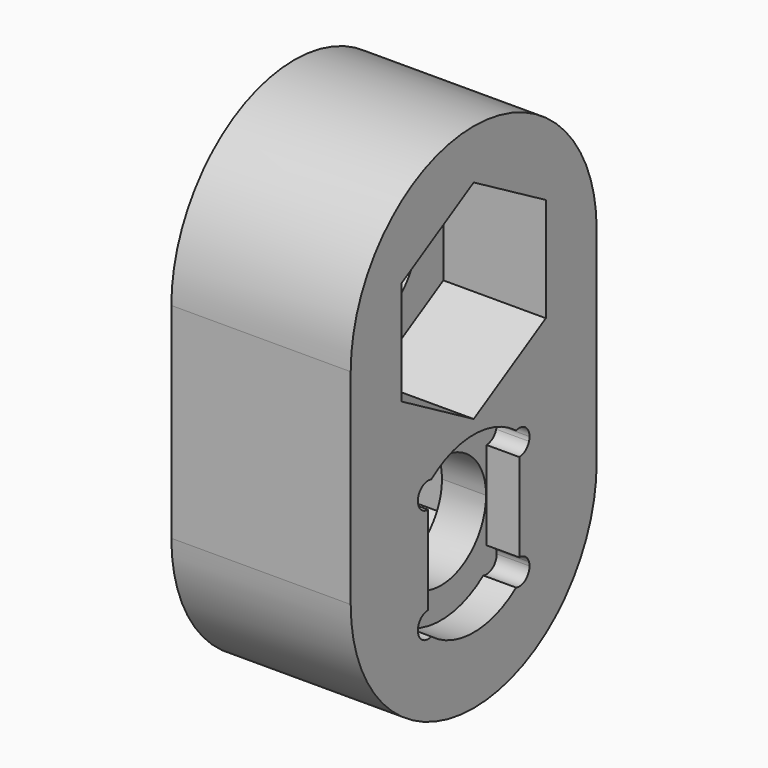
from build123d import *

# Parameters (mm, degrees)
F1_DEPTH = 5.55752
F2_R     = 1.75
F3_DEPTH = 1.016
F4_R     = 1.75
F5_DEPTH = 1.016
F6_DEPTH = 3.175
F7_DEPTH = 3.175


# Not quite as in the source:
# - a feature names something its author has since deleted; it is built from what else it names


with BuildPart() as f1:
    # F0 (on Right) → F1 (new body)
    with BuildSketch(Plane.YZ):
        with BuildLine():
            ThreePointArc((0.636344373, -4.7197957677), (2.2310225415, -4.2076055743), (3.5497579143, -3.175))
            ThreePointArc((3.5497579143, -3.175), (2.2310225415, -2.1423944257), (0.636344373, -1.6302042323))
            ThreePointArc((0.636344373, -1.6302042323), (0, -1.75), (-0.636344373, -1.6302042323))
            ThreePointArc((-0.636344373, -1.6302042323), (-2.2310225415, -2.1423944257), (-3.5497579143, -3.175))
            ThreePointArc((-3.5497579143, -3.175), (-2.2310225415, -4.2076055743), (-0.636344373, -4.7197957677))
            ThreePointArc((-0.636344373, -4.7197957677), (0, -4.6), (0.636344373, -4.7197957677))
        make_face()
        with BuildLine():
            ThreePointArc((3.5497579143, -3.175), (4.4489958596, -1.6993652025), (4.7625, 0))
            ThreePointArc((4.7625, 0), (0, 4.7625), (-4.7625, 0))
            ThreePointArc((-4.7625, 0), (-4.4489958596, -1.6993652025), (-3.5497579143, -3.175))
            ThreePointArc((-3.5497579143, -3.175), (-2.2310225415, -2.1423944257), (-0.636344373, -1.6302042323))
            ThreePointArc((-0.636344373, -1.6302042323), (-0.9871416685, 1.4450091094), (1.75, 0))
            ThreePointArc((1.75, 0), (1.4450091094, -0.9871416685), (0.636344373, -1.6302042323))
            ThreePointArc((0.636344373, -1.6302042323), (2.2310225415, -2.1423944257), (3.5497579143, -3.175))
        make_face()
        with BuildLine():
            Line((4.7625, -6.35), (4.7625, 0))
            ThreePointArc((4.7625, 0), (4.4489958596, -1.6993652025), (3.5497579143, -3.175))
            ThreePointArc((3.5497579143, -3.175), (4.4489958596, -4.6506347975), (4.7625, -6.35))
        make_face()
        with BuildLine():
            ThreePointArc((4.7625, -6.35), (4.4489958596, -4.6506347975), (3.5497579143, -3.175))
            ThreePointArc((3.5497579143, -3.175), (2.2310225415, -4.2076055743), (0.636344373, -4.7197957677))
            ThreePointArc((0.636344373, -4.7197957677), (1.4450091094, -5.3628583315), (1.75, -6.35))
            ThreePointArc((1.75, -6.35), (-0.9871416685, -7.7950091094), (-0.636344373, -4.7197957677))
            ThreePointArc((-0.636344373, -4.7197957677), (-2.2310225415, -4.2076055743), (-3.5497579143, -3.175))
            ThreePointArc((-3.5497579143, -3.175), (-4.4489958596, -4.6506347975), (-4.7625, -6.35))
            ThreePointArc((-4.7625, -6.35), (0, -11.1125), (4.7625, -6.35))
        make_face()
        with BuildLine():
            ThreePointArc((-3.5497579143, -3.175), (-4.4489958596, -1.6993652025), (-4.7625, 0))
            Line((-4.7625, 0), (-4.7625, -6.35))
            ThreePointArc((-4.7625, -6.35), (-4.4489958596, -4.6506347975), (-3.5497579143, -3.175))
        make_face()
    extrude(amount=F1_DEPTH)

    # F2 (on face) → F3 (cut)
    with BuildSketch(Plane.YZ.offset(5.55752)):
        with BuildLine():
            ThreePointArc((1.368425, -4.5847), (1.4846669962, -4.8653330038), (1.7653, -4.981575))
            Line((1.7653, -4.981575), (1.7653, -4.5847))
            Line((1.7653, -4.5847), (1.368425, -4.5847))
        make_face()
        with BuildLine():
            Line((1.7653, -4.5847), (1.7653, -4.981575))
            ThreePointArc((1.7653, -4.981575), (1.9986038099, -4.9057593371), (2.1427708235, -4.7072787218))
            ThreePointArc((2.1427708235, -4.7072787218), (1.9091883092, -4.4408116908), (1.6427212782, -4.2072291765))
            ThreePointArc((1.6427212782, -4.2072291765), (1.4442406629, -4.3513961901), (1.368425, -4.5847))
            Line((1.368425, -4.5847), (1.7653, -4.5847))
        make_face()
        with BuildLine():
            ThreePointArc((1.7653, -7.718425), (1.4846669962, -7.8346669962), (1.368425, -8.1153))
            Line((1.368425, -8.1153), (1.7653, -8.1153))
            Line((1.7653, -8.1153), (1.7653, -7.718425))
        make_face()
        with BuildLine():
            Line((1.7653, -8.1153), (1.368425, -8.1153))
            ThreePointArc((1.368425, -8.1153), (1.4442406629, -8.3486038099), (1.6427212782, -8.4927708235))
            ThreePointArc((1.6427212782, -8.4927708235), (1.9091883092, -8.2591883092), (2.1427708235, -7.9927212782))
            ThreePointArc((2.1427708235, -7.9927212782), (1.9986038099, -7.7942406629), (1.7653, -7.718425))
            Line((1.7653, -7.718425), (1.7653, -8.1153))
        make_face()
        with BuildLine():
            Line((-1.368425, -8.1153), (-1.7653, -8.1153))
            Line((-1.7653, -8.1153), (-1.7653, -7.718425))
            ThreePointArc((-1.7653, -7.718425), (-1.9986038099, -7.7942406629), (-2.1427708235, -7.9927212782))
            ThreePointArc((-2.1427708235, -7.9927212782), (-1.9091883092, -8.2591883092), (-1.6427212782, -8.4927708235))
            ThreePointArc((-1.6427212782, -8.4927708235), (-1.4442406629, -8.3486038099), (-1.368425, -8.1153))
        make_face()
        with BuildLine():
            Line((-1.7653, -7.718425), (-1.7653, -8.1153))
            Line((-1.7653, -8.1153), (-1.368425, -8.1153))
            ThreePointArc((-1.368425, -8.1153), (-1.4846669962, -7.8346669962), (-1.7653, -7.718425))
        make_face()
        with BuildLine():
            Line((-1.7653, -4.5847), (-1.7653, -4.981575))
            ThreePointArc((-1.7653, -4.981575), (-1.4846669962, -4.8653330038), (-1.368425, -4.5847))
            Line((-1.368425, -4.5847), (-1.7653, -4.5847))
        make_face()
        with BuildLine():
            ThreePointArc((-2.1427708235, -4.7072787218), (-1.9986038099, -4.9057593371), (-1.7653, -4.981575))
            Line((-1.7653, -4.981575), (-1.7653, -4.5847))
            Line((-1.7653, -4.5847), (-1.368425, -4.5847))
            ThreePointArc((-1.368425, -4.5847), (-1.4442406629, -4.3513961901), (-1.6427212782, -4.2072291765))
            ThreePointArc((-1.6427212782, -4.2072291765), (-1.9091883092, -4.4408116908), (-2.1427708235, -4.7072787218))
        make_face()
        with BuildLine():
            ThreePointArc((-1.7653, -7.718425), (-1.4846669962, -7.8346669962), (-1.368425, -8.1153))
            Line((-1.368425, -8.1153), (1.368425, -8.1153))
            ThreePointArc((1.368425, -8.1153), (1.4846669962, -7.8346669962), (1.7653, -7.718425))
            Line((1.7653, -7.718425), (1.7653, -4.981575))
            ThreePointArc((1.7653, -4.981575), (1.4846669962, -4.8653330038), (1.368425, -4.5847))
            Line((1.368425, -4.5847), (-1.368425, -4.5847))
            ThreePointArc((-1.368425, -4.5847), (-1.4846669962, -4.8653330038), (-1.7653, -4.981575))
            Line((-1.7653, -4.981575), (-1.7653, -7.718425))
        make_face()
        with Locations((0, -6.35)):
            Circle(F2_R, mode=Mode.SUBTRACT)
        with BuildLine():
            ThreePointArc((-1.6427212782, -4.2072291765), (-2.0459330038, -4.3040669962), (-2.1427708235, -4.7072787218))
            ThreePointArc((-2.1427708235, -4.7072787218), (-1.9091883092, -4.4408116908), (-1.6427212782, -4.2072291765))
        make_face()
        with BuildLine():
            ThreePointArc((1.6427212782, -4.2072291765), (1.9091883092, -4.4408116908), (2.1427708235, -4.7072787218))
            ThreePointArc((2.1427708235, -4.7072787218), (2.1572939405, -4.6467525283), (2.162175, -4.5847))
            ThreePointArc((2.162175, -4.5847), (1.9986038099, -4.2636406629), (1.6427212782, -4.2072291765))
        make_face()
        with BuildLine():
            ThreePointArc((2.1427708235, -7.9927212782), (1.9091883092, -8.2591883092), (1.6427212782, -8.4927708235))
            ThreePointArc((1.6427212782, -8.4927708235), (1.9986038099, -8.4363593371), (2.162175, -8.1153))
            ThreePointArc((2.162175, -8.1153), (2.1572939405, -8.0532474717), (2.1427708235, -7.9927212782))
        make_face()
        with BuildLine():
            ThreePointArc((-2.1427708235, -7.9927212782), (-2.0459330038, -8.3959330038), (-1.6427212782, -8.4927708235))
            ThreePointArc((-1.6427212782, -8.4927708235), (-1.9091883092, -8.2591883092), (-2.1427708235, -7.9927212782))
        make_face()
        with BuildLine():
            ThreePointArc((-1.6427212782, -4.2072291765), (-1.4442406629, -4.3513961901), (-1.368425, -4.5847))
            Line((-1.368425, -4.5847), (1.368425, -4.5847))
            ThreePointArc((1.368425, -4.5847), (1.4442406629, -4.3513961901), (1.6427212782, -4.2072291765))
            ThreePointArc((1.6427212782, -4.2072291765), (0, -3.65), (-1.6427212782, -4.2072291765))
        make_face()
        with BuildLine():
            Line((1.368425, -8.1153), (-1.368425, -8.1153))
            ThreePointArc((-1.368425, -8.1153), (-1.4442406629, -8.3486038099), (-1.6427212782, -8.4927708235))
            ThreePointArc((-1.6427212782, -8.4927708235), (0, -9.05), (1.6427212782, -8.4927708235))
            ThreePointArc((1.6427212782, -8.4927708235), (1.4442406629, -8.3486038099), (1.368425, -8.1153))
        make_face()
    extrude(amount=-F3_DEPTH, mode=Mode.SUBTRACT)

    # F4 (on face) → F5 (cut)
    with BuildSketch(Plane(origin=(0, 0, 0), x_dir=(0, -1, 0), z_dir=(-1, 0, 0))):
        with BuildLine():
            ThreePointArc((1.7653, -1.368425), (1.4846669962, -1.4846669962), (1.368425, -1.7653))
            Line((1.368425, -1.7653), (1.7653, -1.7653))
            Line((1.7653, -1.7653), (1.7653, -1.368425))
        make_face()
        with BuildLine():
            Line((1.7653, -1.7653), (1.368425, -1.7653))
            ThreePointArc((1.368425, -1.7653), (1.4442406629, -1.9986038099), (1.6427212782, -2.1427708235))
            ThreePointArc((1.6427212782, -2.1427708235), (1.9091883092, -1.9091883092), (2.1427708235, -1.6427212782))
            ThreePointArc((2.1427708235, -1.6427212782), (1.9986038099, -1.4442406629), (1.7653, -1.368425))
            Line((1.7653, -1.368425), (1.7653, -1.7653))
        make_face()
        with BuildLine():
            Line((-1.7653, -1.368425), (-1.7653, -1.7653))
            Line((-1.7653, -1.7653), (-1.368425, -1.7653))
            ThreePointArc((-1.368425, -1.7653), (-1.4846669962, -1.4846669962), (-1.7653, -1.368425))
        make_face()
        with BuildLine():
            Line((-1.368425, -1.7653), (-1.7653, -1.7653))
            Line((-1.7653, -1.7653), (-1.7653, -1.368425))
            ThreePointArc((-1.7653, -1.368425), (-1.9986038099, -1.4442406629), (-2.1427708235, -1.6427212782))
            ThreePointArc((-2.1427708235, -1.6427212782), (-1.9091883092, -1.9091883092), (-1.6427212782, -2.1427708235))
            ThreePointArc((-1.6427212782, -2.1427708235), (-1.4442406629, -1.9986038099), (-1.368425, -1.7653))
        make_face()
        with BuildLine():
            Line((-1.7653, 1.7653), (-1.7653, 1.368425))
            ThreePointArc((-1.7653, 1.368425), (-1.4846669962, 1.4846669962), (-1.368425, 1.7653))
            Line((-1.368425, 1.7653), (-1.7653, 1.7653))
        make_face()
        with BuildLine():
            ThreePointArc((-2.1427708235, 1.6427212782), (-1.9986038099, 1.4442406629), (-1.7653, 1.368425))
            Line((-1.7653, 1.368425), (-1.7653, 1.7653))
            Line((-1.7653, 1.7653), (-1.368425, 1.7653))
            ThreePointArc((-1.368425, 1.7653), (-1.4442406629, 1.9986038099), (-1.6427212782, 2.1427708235))
            ThreePointArc((-1.6427212782, 2.1427708235), (-1.9091883092, 1.9091883092), (-2.1427708235, 1.6427212782))
        make_face()
        with BuildLine():
            ThreePointArc((1.368425, 1.7653), (1.4846669962, 1.4846669962), (1.7653, 1.368425))
            Line((1.7653, 1.368425), (1.7653, 1.7653))
            Line((1.7653, 1.7653), (1.368425, 1.7653))
        make_face()
        with BuildLine():
            Line((1.7653, 1.7653), (1.7653, 1.368425))
            ThreePointArc((1.7653, 1.368425), (1.9986038099, 1.4442406629), (2.1427708235, 1.6427212782))
            ThreePointArc((2.1427708235, 1.6427212782), (1.9091883092, 1.9091883092), (1.6427212782, 2.1427708235))
            ThreePointArc((1.6427212782, 2.1427708235), (1.4442406629, 1.9986038099), (1.368425, 1.7653))
            Line((1.368425, 1.7653), (1.7653, 1.7653))
        make_face()
        with BuildLine():
            ThreePointArc((-1.7653, -1.368425), (-1.4846669962, -1.4846669962), (-1.368425, -1.7653))
            Line((-1.368425, -1.7653), (1.368425, -1.7653))
            ThreePointArc((1.368425, -1.7653), (1.4846669962, -1.4846669962), (1.7653, -1.368425))
            Line((1.7653, -1.368425), (1.7653, 1.368425))
            ThreePointArc((1.7653, 1.368425), (1.4846669962, 1.4846669962), (1.368425, 1.7653))
            Line((1.368425, 1.7653), (-1.368425, 1.7653))
            ThreePointArc((-1.368425, 1.7653), (-1.4846669962, 1.4846669962), (-1.7653, 1.368425))
            Line((-1.7653, 1.368425), (-1.7653, -1.368425))
        make_face()
        Circle(F4_R, mode=Mode.SUBTRACT)
        with BuildLine():
            ThreePointArc((-1.6427212782, 2.1427708235), (-2.0459330038, 2.0459330038), (-2.1427708235, 1.6427212782))
            ThreePointArc((-2.1427708235, 1.6427212782), (-1.9091883092, 1.9091883092), (-1.6427212782, 2.1427708235))
        make_face()
        with BuildLine():
            ThreePointArc((1.6427212782, 2.1427708235), (1.9091883092, 1.9091883092), (2.1427708235, 1.6427212782))
            ThreePointArc((2.1427708235, 1.6427212782), (2.1572939405, 1.7032474717), (2.162175, 1.7653))
            ThreePointArc((2.162175, 1.7653), (1.9986038099, 2.0863593371), (1.6427212782, 2.1427708235))
        make_face()
        with BuildLine():
            ThreePointArc((2.1427708235, -1.6427212782), (1.9091883092, -1.9091883092), (1.6427212782, -2.1427708235))
            ThreePointArc((1.6427212782, -2.1427708235), (1.9986038099, -2.0863593371), (2.162175, -1.7653))
            ThreePointArc((2.162175, -1.7653), (2.1572939405, -1.7032474717), (2.1427708235, -1.6427212782))
        make_face()
        with BuildLine():
            ThreePointArc((-2.1427708235, -1.6427212782), (-2.0459330038, -2.0459330038), (-1.6427212782, -2.1427708235))
            ThreePointArc((-1.6427212782, -2.1427708235), (-1.9091883092, -1.9091883092), (-2.1427708235, -1.6427212782))
        make_face()
        with BuildLine():
            ThreePointArc((-1.6427212782, 2.1427708235), (-1.4442406629, 1.9986038099), (-1.368425, 1.7653))
            Line((-1.368425, 1.7653), (1.368425, 1.7653))
            ThreePointArc((1.368425, 1.7653), (1.4442406629, 1.9986038099), (1.6427212782, 2.1427708235))
            ThreePointArc((1.6427212782, 2.1427708235), (0, 2.7), (-1.6427212782, 2.1427708235))
        make_face()
        with BuildLine():
            Line((1.368425, -1.7653), (-1.368425, -1.7653))
            ThreePointArc((-1.368425, -1.7653), (-1.4442406629, -1.9986038099), (-1.6427212782, -2.1427708235))
            ThreePointArc((-1.6427212782, -2.1427708235), (0, -2.7), (1.6427212782, -2.1427708235))
            ThreePointArc((1.6427212782, -2.1427708235), (1.4442406629, -1.9986038099), (1.368425, -1.7653))
        make_face()
    extrude(amount=-F5_DEPTH, mode=Mode.SUBTRACT)

    # F2 (on face) → F6 (cut)
    with BuildSketch(Plane.YZ.offset(5.55752)):
        Polygon((-2.794, -1.6131166521), (0, -3.2262333042), (2.794, -1.6131166521), (2.794, 1.6131166521), (0, 3.2262333042), (-2.794, 1.6131166521), align=None)
        Circle(F2_R, mode=Mode.SUBTRACT)
    extrude(amount=-F6_DEPTH, mode=Mode.SUBTRACT)

    # F4 (on face) → F7 (cut)
    with BuildSketch(Plane(origin=(0, 0, 0), x_dir=(0, -1, 0), z_dir=(-1, 0, 0))):
        Polygon((-2.794, -7.9631166521), (0, -9.5762333042), (2.794, -7.9631166521), (2.794, -4.7368833479), (0, -3.1237666958), (-2.794, -4.7368833479), align=None)
        with Locations((0, -6.35)):
            Circle(F4_R, mode=Mode.SUBTRACT)
    extrude(amount=-F7_DEPTH, mode=Mode.SUBTRACT)


solid = f1.part
